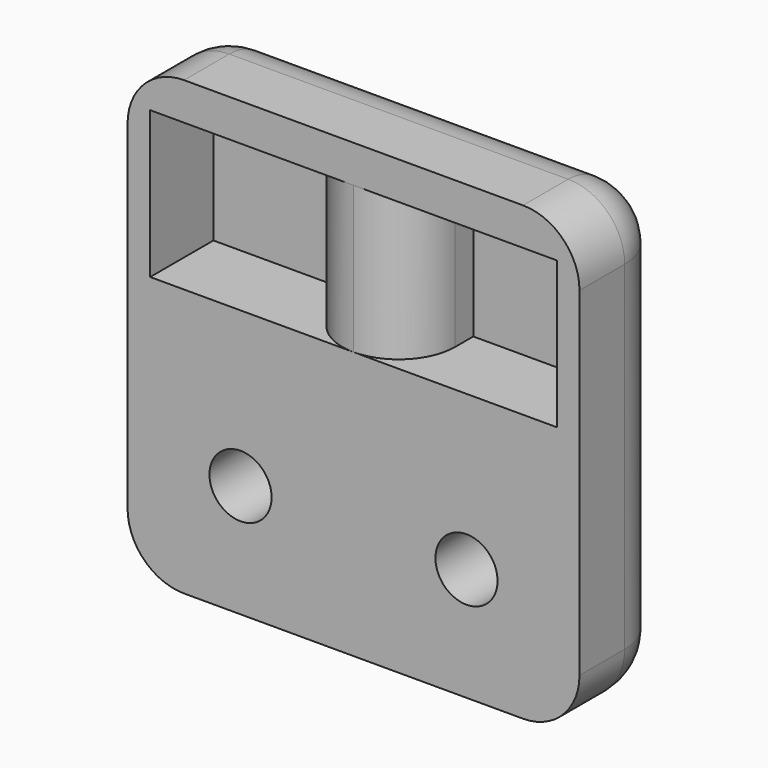
from build123d import *

# Parameters (mm, degrees)
F0_W     = 40
F0_H     = 40
F0_W_2   = 13
F0_H_2   = 13
F1_DEPTH = 10
F2_DEPTH = 7
F0_W_3   = 10
F3_DEPTH = 10
F4_R     = 4.99999
F5_R     = 5
F6_D     = 5.5
F6_DEPTH = 7
F6_TIP   = 1.6523667023


# Not quite as in the source:
# - a fillet or chamfer is up to 0.001 mm smaller than in the source, because OpenCascade refuses the exact size
# - a feature names something its author has since deleted; it is built from what else it names


with BuildPart() as f1:
    # F0 (on Front) → F1 (new body)
    with BuildSketch(Plane.XZ):
        Rectangle(F0_W, F0_H)
        Polygon((-18, 3.6852569133), (-18, 16.6852569133), (-5, 16.6852569133), (5, 16.6852569133), (18, 16.6852569133), (18, 3.6852569133), (5, 3.6852569133), (-5, 3.6852569133), align=None, mode=Mode.SUBTRACT)
        with Locations((-11.5, 10.1852569133)):
            Rectangle(F0_W_2, F0_H_2)
        with Locations((11.5, 10.1852569133)):
            Rectangle(F0_W_2, F0_H_2)
    extrude(amount=-F1_DEPTH)

    # F0 (on Front) → F2 (cut)
    with BuildSketch(Plane.XZ):
        with Locations((-11.5, 10.1852569133)):
            Rectangle(F0_W_2, F0_H_2)
        with Locations((11.5, 10.1852569133)):
            Rectangle(F0_W_2, F0_H_2)
    extrude(amount=-F2_DEPTH, mode=Mode.SUBTRACT)

    # F0 (on Front) → F3 (join)
    with BuildSketch(Plane.XZ):
        with Locations((0, 10.1852569133)):
            Rectangle(F0_W_3, F0_H_2)
    extrude(amount=-F3_DEPTH)

    # F4 (radius 5 in the source; OpenCascade refuses exactly that, so slightly less here)
    f4_edges = [f1.edges().sort_by_distance(p)[0] for p in [
        (5, 0, 10.185257),
        (-5, 0, 10.185257),
    ]]
    fillet(f4_edges, radius=F4_R)

    # F5
    f5_edges = [f1.edges().sort_by_distance(p)[0] for p in [
        (0, 10, 20),
        (20, 5, 20),
        (-20, 5, 20),
        (20, 5, -20),
        (0, 10, -20),
        (-20, 5, -20),
        (-20, 10, 0),
        (20, 10, 0),
    ]]
    fillet(f5_edges, radius=F5_R)

    # F6
    with Locations(Plane.XZ):
        with Locations((-10, -10), (10, -10)):
            Hole(F6_D / 2, depth=F6_DEPTH)
            with Locations((0, 0, -(F6_DEPTH + F6_TIP / 2))):  # 118° drill point
                Cone(0, F6_D / 2, F6_TIP, mode=Mode.SUBTRACT)


solid = f1.part
